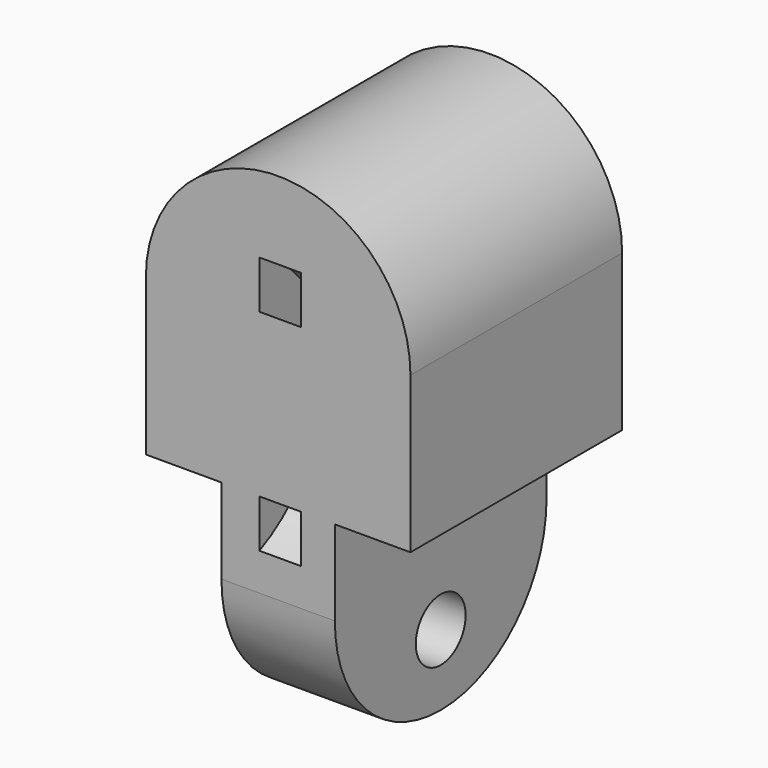
from build123d import *

# Parameters (mm, degrees)
F1_DEPTH  = 14
F2_R      = 1.65
F3_DEPTH  = 25
F4_R      = 6.99999
F5_R      = 1.125
F7_R      = 1.125
F9_W      = 14
F9_H      = 6.4348620027
F10_DEPTH = 29.7
F13_DEPTH = 1.1


# Not quite as in the source:
# - a fillet or chamfer is up to 0.001 mm smaller than in the source, because OpenCascade refuses the exact size


with BuildPart() as f1:
    # F0 (on Front) → F1 (new body)
    with BuildSketch(Plane.XZ):
        with BuildLine():
            ThreePointArc((-24.6100064665, 31.2714347113), (-31.6100064665, 38.2714347113), (-38.6100064665, 31.2714347113))
            Line((-38.6100064665, 31.2714347113), (-38.6100064665, 23.0214347113))
            Line((-38.6100064665, 23.0214347113), (-34.6100064665, 23.0214347113))
            Line((-34.6100064665, 23.0214347113), (-34.6100064665, 22.0214347113))
            Line((-34.6100064665, 22.0214347113), (-34.6100064665, 19.0214347113))
            Line((-34.6100064665, 19.0214347113), (-34.6100064665, 11.5214347113))
            Line((-34.6100064665, 11.5214347113), (-28.6100064665, 11.5214347113))
            Line((-28.6100064665, 11.5214347113), (-28.6100064665, 15.2714347113))
            Line((-28.6100064665, 15.2714347113), (-28.6100064665, 19.0214347113))
            Line((-28.6100064665, 19.0214347113), (-28.6100064665, 22.0214347113))
            Line((-28.6100064665, 22.0214347113), (-28.6100064665, 23.0214347113))
            Line((-28.6100064665, 23.0214347113), (-24.6100064665, 23.0214347113))
            Line((-24.6100064665, 23.0214347113), (-24.6100064665, 31.2714347113))
        make_face()
    extrude(amount=F1_DEPTH)

    # F2 (on face) → F3 (cut)
    with BuildSketch(Plane.YZ.offset(-28.6100064665)):
        with Locations((-7, 15.2714347113)):
            Circle(F2_R)
    extrude(amount=-F3_DEPTH, mode=Mode.SUBTRACT)

    # F4 (radius 7 in the source; OpenCascade refuses exactly that, so slightly less here)
    f4_edges = [f1.edges().sort_by_distance(p)[0] for p in [
        (-31.610006, -14, 11.521435),
        (-31.610006, 0, 11.521435),
    ]]
    fillet(f4_edges, radius=F4_R)

    # F5 (on face) → F6 (revolve)
    with BuildSketch(Plane.XZ.offset(14)):
        with Locations((-34.6100064665, 27.1464347113)):
            Circle(F5_R)
    revolve(axis=Axis((-31.6100064665, -14, 28.3964347113), (0, 0, -1)))

    # F7 (on face) → F8 (revolve)
    with BuildSketch(Plane(origin=(0, 0, 0), x_dir=(-1, 0, 0), z_dir=(0, 1, 0))):
        with Locations((28.6100064665, 27.1464347113)):
            Circle(F7_R)
    revolve(axis=Axis((-31.6100064665, 0, 28.3964347113), (0, 0, -1)))

    # F9 (on Top) → F10 (cut)
    with BuildSketch(Plane.XY):
        with Locations((-31.6100064665, -17.2174310014)):
            Rectangle(F9_W, F9_H)
    extrude(amount=F10_DEPTH, mode=Mode.SUBTRACT)

    # F12 (on offset) → F13 (cut, symmetric)
    with BuildSketch(Plane.YZ.offset(-31.5)):
        with BuildLine():
            ThreePointArc((-14, 31.6231168223), (-11.8, 27.3242797703), (-14, 23.0254427182))
            Line((-14, 23.0254427182), (-14, 20.4949313387))
            ThreePointArc((-14, 20.4949313387), (-9.6, 27.3242797703), (-14, 34.1536282018))
            Line((-14, 34.1536282018), (-14, 31.6231168223))
        make_face()
    extrude(amount=F13_DEPTH, both=True, mode=Mode.SUBTRACT)


solid = f1.part
